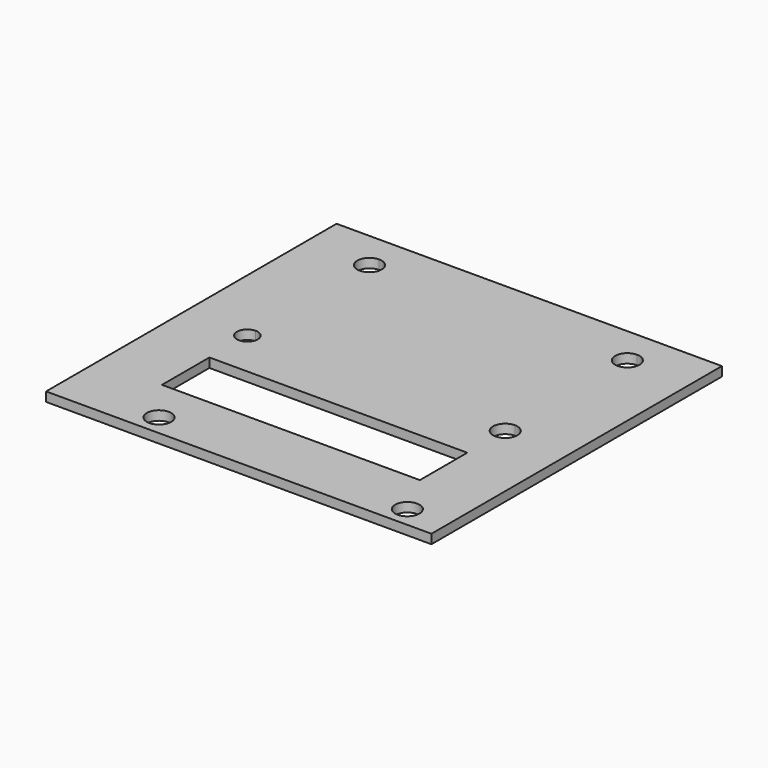
from build123d import *

# Parameters (mm, degrees)
F1_DEPTH = 1.5875


# Not quite as in the source:
# - a length typed as a fraction of an inch, garbled in the dataset ("3 / 203.2 mm" for 3/8 in), is restored


with BuildPart() as f1:
    # F0 (on Top) → F1 (new body)
    with BuildSketch(Plane.XY):
        with BuildLine():
            Line((22.098, 26.5938), (22.098, 31.115))
            Line((22.098, 31.115), (0, 31.115))
            Line((0, 31.115), (-22.098, 31.115))
            Line((-22.098, 31.115), (-22.098, 26.5938))
            ThreePointArc((-22.098, 26.5938), (-20.6252379961, 25.9837620039), (-20.0152, 24.511))
            ThreePointArc((-20.0152, 24.511), (-20.6252379961, 23.0382379961), (-22.098, 22.4282))
            Line((-22.098, 22.4282), (-22.098, 0.127))
            ThreePointArc((-22.098, 0.127), (-20.8407641431, -0.3937641431), (-20.32, -1.651))
            ThreePointArc((-20.32, -1.651), (-20.8407641431, -2.9082358569), (-22.098, -3.429))
            Line((-22.098, -3.429), (-22.098, -9.779))
            Line((-22.098, -9.779), (22.098, -9.779))
            Line((22.098, -9.779), (22.098, -3.7338))
            ThreePointArc((22.098, -3.7338), (20.0152, -1.651), (22.098, 0.4318))
            Line((22.098, 0.4318), (22.098, 22.4282))
            ThreePointArc((22.098, 22.4282), (20.0152, 24.511), (22.098, 26.5938))
        make_face()
        with BuildLine():
            Line((-22.098, 26.5938), (-22.098, 31.115))
            Line((-22.098, 31.115), (-33.02, 31.115))
            Line((-33.02, 31.115), (-33.02, -31.115))
            Line((-33.02, -31.115), (-22.098, -31.115))
            Line((-22.098, -31.115), (-22.098, -27.559))
            Line((-22.098, -27.559), (-22.098, -19.939))
            Line((-22.098, -19.939), (-22.098, -9.779))
            Line((-22.098, -9.779), (-22.098, -3.429))
            ThreePointArc((-22.098, -3.429), (-23.876, -1.651), (-22.098, 0.127))
            Line((-22.098, 0.127), (-22.098, 22.4282))
            ThreePointArc((-22.098, 22.4282), (-24.1808, 24.511), (-22.098, 26.5938))
        make_face()
        with BuildLine():
            Line((33.02, -27.559), (33.02, 31.115))
            Line((33.02, 31.115), (22.098, 31.115))
            Line((22.098, 31.115), (22.098, 26.5938))
            ThreePointArc((22.098, 26.5938), (23.5707620039, 25.9837620039), (24.1808, 24.511))
            ThreePointArc((24.1808, 24.511), (23.5707620039, 23.0382379961), (22.098, 22.4282))
            Line((22.098, 22.4282), (22.098, 0.4318))
            ThreePointArc((22.098, 0.4318), (23.5707620039, -0.1782379961), (24.1808, -1.651))
            ThreePointArc((24.1808, -1.651), (23.5707620039, -3.1237620039), (22.098, -3.7338))
            Line((22.098, -3.7338), (22.098, -9.779))
            Line((22.098, -9.779), (22.098, -19.939))
            Line((22.098, -19.939), (22.098, -27.559))
            Line((22.098, -27.559), (23.9649, -27.559))
            ThreePointArc((23.9649, -27.559), (26.0477, -25.4762), (28.1305, -27.559))
            Line((28.1305, -27.559), (33.02, -27.559))
        make_face()
        with BuildLine():
            Line((33.02, -31.115), (33.02, -27.559))
            Line((33.02, -27.559), (28.1305, -27.559))
            ThreePointArc((28.1305, -27.559), (26.0477, -29.6418), (23.9649, -27.559))
            Line((23.9649, -27.559), (22.098, -27.559))
            Line((22.098, -27.559), (22.098, -31.115))
            Line((22.098, -31.115), (33.02, -31.115))
        make_face()
        with BuildLine():
            Line((-14.4272, -27.559), (22.098, -27.559))
            Line((22.098, -27.559), (22.098, -19.939))
            Line((22.098, -19.939), (-22.098, -19.939))
            Line((-22.098, -19.939), (-22.098, -27.559))
            Line((-22.098, -27.559), (-18.5928, -27.559))
            ThreePointArc((-18.5928, -27.559), (-16.51, -25.4762), (-14.4272, -27.559))
        make_face()
        with BuildLine():
            Line((-22.098, -31.115), (22.098, -31.115))
            Line((22.098, -31.115), (22.098, -27.559))
            Line((22.098, -27.559), (-14.4272, -27.559))
            ThreePointArc((-14.4272, -27.559), (-16.51, -29.6418), (-18.5928, -27.559))
            Line((-18.5928, -27.559), (-22.098, -27.559))
            Line((-22.098, -27.559), (-22.098, -31.115))
        make_face()
    extrude(amount=F1_DEPTH)


solid = f1.part
